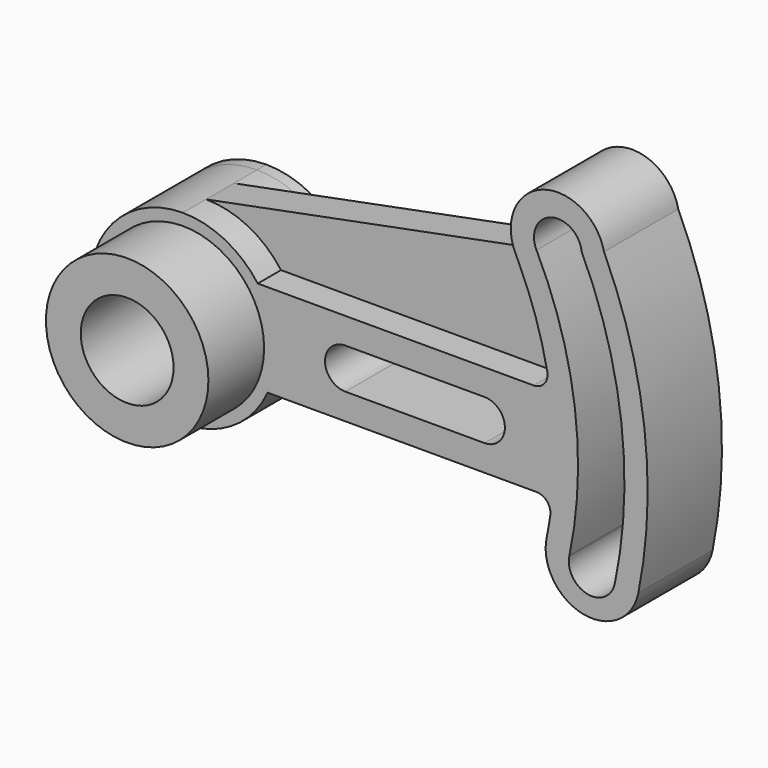
from build123d import *

# Parameters (mm, degrees)
F0_R     = 22.225
F0_R_2   = 12.7
F1_DEPTH = 25.4
F2_DEPTH = 44.45
F3_DEPTH = 3.175
F4_DEPTH = 17.4498
F5_DEPTH = 7.9248


with BuildPart() as f1:
    # F0 (on Front) → F1 (new body)
    with BuildSketch(Plane.XZ):
        with BuildLine():
            Line((28.6733515832, 12.7), (-43.0187255819, 12.7))
            ThreePointArc((-43.0187255819, 12.7), (-39.3609821014, 5.5810953524), (-38.1, -2.3225629708))
            ThreePointArc((-38.1, -2.3225629708), (-38.6603373258, -7.6283294781), (-40.3166266323, -12.7))
            Line((-40.3166266323, -12.7), (28.6733515832, -12.7))
            Line((28.6733515832, -12.7), (33.2553653837, -12.7))
            ThreePointArc((33.2553653837, -12.7), (36.1382550159, -14.0190067506), (37.0250549441, -17.0627572869))
            ThreePointArc((37.0250549441, -17.0627572869), (36.5597775982, -19.9464361831), (36.0117960852, -22.8155481096))
            ThreePointArc((36.0117960852, -22.8155481096), (45.993088379, -37.9530956056), (61.1179671118, -27.9526164488))
            ThreePointArc((61.1179671118, -27.9526164488), (62.7752437383, 12.3436674732), (51.7147344593, 51.1277131392))
            ThreePointArc((51.7147344593, 51.1277131392), (34.8831774474, 60.656419548), (27.5508360528, 42.7585334455))
            ThreePointArc((27.5508360528, 42.7585334455), (27.9929024003, 41.8544537956), (28.4259920573, 40.9460397831))
            ThreePointArc((28.4259920573, 40.9460397831), (33.0422300736, 29.3343132556), (36.198144095, 17.2437362196))
            ThreePointArc((36.198144095, 17.2437362196), (35.4015407636, 14.0891979632), (32.4594636915, 12.7))
            Line((32.4594636915, 12.7), (28.6733515832, 12.7))
        make_face()
        with BuildLine():
            Line((-19.05, 5.5499), (19.05, 5.5499))
            ThreePointArc((19.05, 5.5499), (24.5999, 0), (19.05, -5.5499))
            Line((19.05, -5.5499), (-19.05, -5.5499))
            ThreePointArc((-19.05, -5.5499), (-24.5999, 0), (-19.05, 5.5499))
        make_face(mode=Mode.SUBTRACT)
        with BuildLine():
            ThreePointArc((45.5992916154, 49.2079816191), (56.4779805656, 11.5237748752), (54.6936829038, -27.6586394588))
            ThreePointArc((54.6936829038, -27.6586394588), (47.3123292859, -32.7813536179), (42.1896151268, -25.4))
            ThreePointArc((42.1896151268, -25.4), (42.2286106989, -25.2021250663), (42.2738673123, -25.0055875814))
            ThreePointArc((42.2738673123, -25.0055875814), (43.7417669199, 11.0404436441), (33.2508024974, 45.5572621802))
            ThreePointArc((33.2508024974, 45.5572621802), (37.2475404836, 54.7479964973), (45.5992916154, 49.2079816191))
        make_face(mode=Mode.SUBTRACT)
        with BuildLine():
            ThreePointArc((-38.1, -2.3225629708), (-39.3609821014, 5.5810953524), (-43.0187255819, 12.7))
            ThreePointArc((-43.0187255819, 12.7), (-52.0198671492, 20.3350306731), (-63.5, 23.0774370292))
            ThreePointArc((-63.5, 23.0774370292), (-84.8160373961, -16.1351134134), (-40.3166266323, -12.7))
            ThreePointArc((-40.3166266323, -12.7), (-38.6603373258, -7.6283294781), (-38.1, -2.3225629708))
        make_face()
        with Locations((-63.5, -2.3225629708)):
            Circle(F0_R, mode=Mode.SUBTRACT)
        with Locations((-63.5, -2.3225629708)):
            Circle(F0_R)
        with Locations((-63.5, -2.3225629708)):
            Circle(F0_R_2, mode=Mode.SUBTRACT)
    extrude(amount=F1_DEPTH)

    # F0 (on Front) → F4 (join)
    with BuildSketch(Plane.XZ):
        with BuildLine():
            ThreePointArc((-63.5, 23.0774370292), (-52.0198671492, 20.3350306731), (-43.0187255819, 12.7))
            Line((-43.0187255819, 12.7), (28.6733515832, 12.7))
            Line((28.6733515832, 12.7), (32.4594636915, 12.7))
            ThreePointArc((32.4594636915, 12.7), (35.4015407636, 14.0891979632), (36.198144095, 17.2437362196))
            ThreePointArc((36.198144095, 17.2437362196), (33.0422300736, 29.3343132556), (28.4259920573, 40.9460397831))
            Line((28.4259920573, 40.9460397831), (-63.5, 23.0774370292))
        make_face()
    extrude(amount=F4_DEPTH)

    # F0 (on Front) → F5 (cut)
    with BuildSketch(Plane.XZ):
        with BuildLine():
            ThreePointArc((-63.5, 23.0774370292), (-52.0198671492, 20.3350306731), (-43.0187255819, 12.7))
            Line((-43.0187255819, 12.7), (28.6733515832, 12.7))
            Line((28.6733515832, 12.7), (32.4594636915, 12.7))
            ThreePointArc((32.4594636915, 12.7), (35.4015407636, 14.0891979632), (36.198144095, 17.2437362196))
            ThreePointArc((36.198144095, 17.2437362196), (33.0422300736, 29.3343132556), (28.4259920573, 40.9460397831))
            Line((28.4259920573, 40.9460397831), (-63.5, 23.0774370292))
        make_face()
    extrude(amount=F5_DEPTH, mode=Mode.SUBTRACT)


with BuildPart() as f2:
    # F0 (on Front) → F2 (new body)
    with BuildSketch(Plane.XZ):
        with Locations((-63.5, -2.3225629708)):
            Circle(F0_R)
        with Locations((-63.5, -2.3225629708)):
            Circle(F0_R_2, mode=Mode.SUBTRACT)
    extrude(amount=F2_DEPTH)


with BuildPart() as f3:
    # F0 (on Front) → F3 (new body)
    with BuildSketch(Plane.XZ):
        with BuildLine():
            ThreePointArc((-38.1, -2.3225629708), (-39.3609821014, 5.5810953524), (-43.0187255819, 12.7))
            ThreePointArc((-43.0187255819, 12.7), (-52.0198671492, 20.3350306731), (-63.5, 23.0774370292))
            ThreePointArc((-63.5, 23.0774370292), (-84.8160373961, -16.1351134134), (-40.3166266323, -12.7))
            ThreePointArc((-40.3166266323, -12.7), (-38.6603373258, -7.6283294781), (-38.1, -2.3225629708))
        make_face()
        with Locations((-63.5, -2.3225629708)):
            Circle(F0_R, mode=Mode.SUBTRACT)
        with Locations((-63.5, -2.3225629708)):
            Circle(F0_R)
        with Locations((-63.5, -2.3225629708)):
            Circle(F0_R_2, mode=Mode.SUBTRACT)
    extrude(amount=-F3_DEPTH)


solid = Compound([f1.part, f2.part, f3.part])
